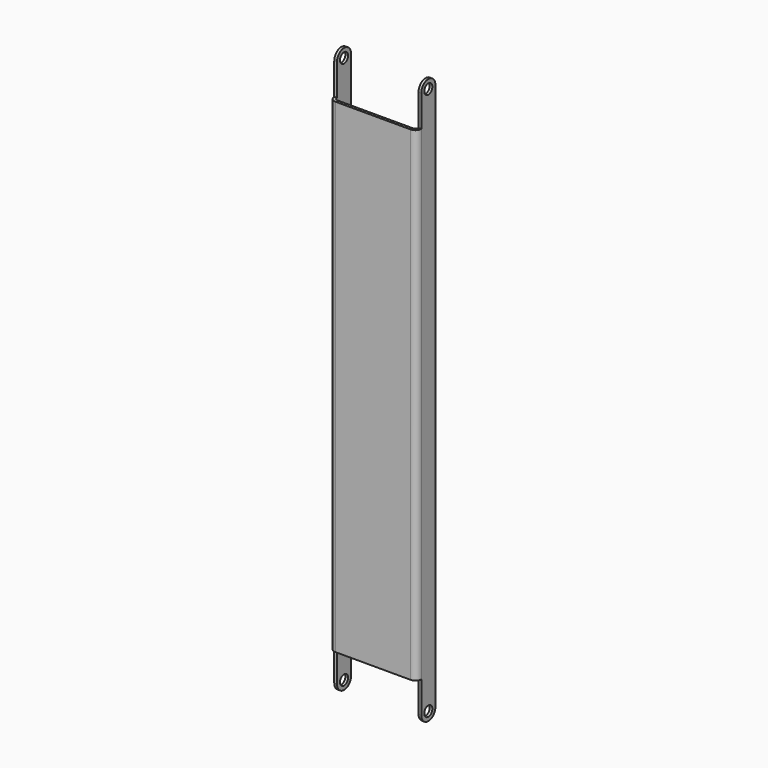
from build123d import *

# Parameters (mm, degrees)
F1_DEPTH = 304.8
F2_R     = 3.69316
F3_R     = 1.98374
F4_W     = 1.70942
F4_H     = 25.4
F6_DEPTH = 11.1125
F7_R     = 5.55624
F8_R     = 3.175
F9_DEPTH = 54.737


# Not quite as in the source:
# - a fillet or chamfer is up to 0.001 mm smaller than in the source, because OpenCascade refuses the exact size


with BuildPart() as f1:
    # F0 (on Top) → F1 (new body)
    with BuildSketch(Plane.XY):
        Polygon((0, 13.09624), (0, 0), (-51.31816, 0), (-51.31816, 13.09624), (-53.02758, 13.09624), (-53.02758, -1.70942), (1.70942, -1.70942), (1.70942, 13.09624), align=None)
    extrude(amount=F1_DEPTH)

    # F2
    f2_edges = [f1.edges().sort_by_distance(p)[0] for p in [
        (1.70942, -1.70942, 152.4),
        (-53.02758, -1.70942, 152.4),
    ]]
    fillet(f2_edges, radius=F2_R)

    # F3
    f3_edges = [f1.edges().sort_by_distance(p)[0] for p in [
        (0, 0, 152.4),
        (-51.31816, 0, 152.4),
    ]]
    fillet(f3_edges, radius=F3_R)

    # F4 (on face) → F6 (join, through all)
    with BuildSketch(Plane(origin=(0, 13.09624, 0), x_dir=(-1, 0, 0), z_dir=(0, 1, 0))):
        with Locations((52.17287, 317.5)):
            Rectangle(F4_W, F4_H)
        with Locations((-0.85471, 317.5)):
            Rectangle(F4_W, F4_H)
        with Locations((-0.85471, -12.7)):
            Rectangle(F4_W, F4_H)
        with Locations((52.17287, -12.7)):
            Rectangle(F4_W, F4_H)
    extrude(amount=-F6_DEPTH)

    # F7 (radius 5.55625 in the source; OpenCascade refuses exactly that, so slightly less here)
    f7_edges = [f1.edges().sort_by_distance(p)[0] for p in [
        (-52.17287, 13.09624, -25.4),
        (0.85471, 13.09624, -25.4),
        (0.85471, 13.09624, 330.2),
        (-52.17287, 13.09624, 330.2),
        (-52.17287, 1.98374, -25.4),
        (-52.17287, 1.98374, 330.2),
        (0.85471, 1.98374, 330.2),
        (0.85471, 1.98374, -25.4),
    ]]
    fillet(f7_edges, radius=F7_R)

    # F8 (on face) → F9 (cut, through all)
    with BuildSketch(Plane.YZ.offset(1.70942)):
        with Locations((7.53999, -19.84375)):
            Circle(F8_R)
        with Locations((7.53999, 324.64375)):
            Circle(F8_R)
    extrude(amount=-F9_DEPTH, mode=Mode.SUBTRACT)


solid = f1.part
